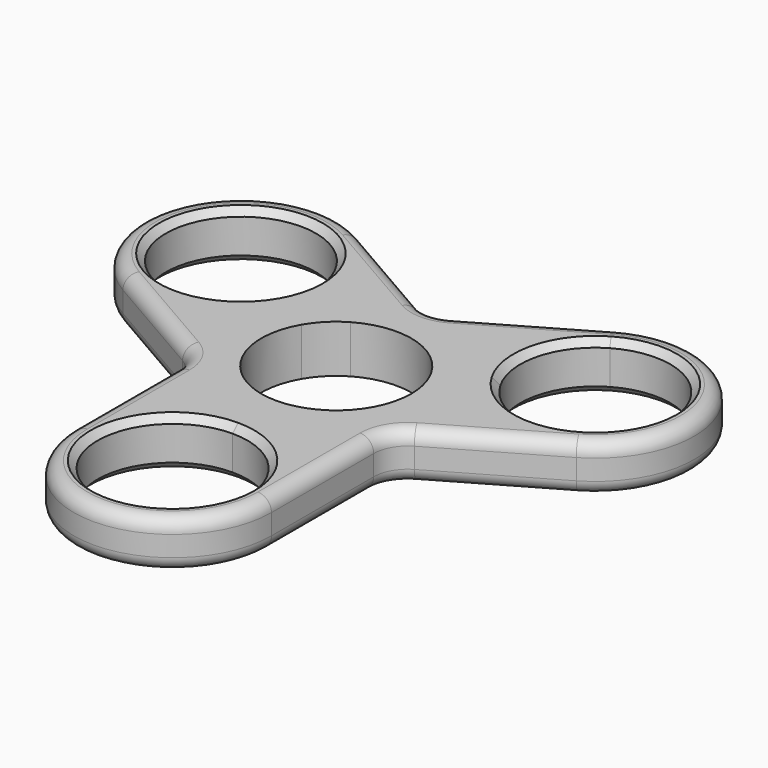
from build123d import *

# Parameters (mm, degrees)
F1_DEPTH    = 7
F3_DEPTH    = 7.001
F5_COUNT    = 3
F7_T1_DEPTH = 7
F8_R        = 2
F9_SIZE     = 1


# Not quite as in the source:
# - a fillet or chamfer that OpenCascade refuses, or shapes differently, is made with other operations: its cross-section is extruded or revolved along the edge and cut away or added
# - a feature names something its author has since deleted; it is built from what else it names


with BuildPart() as f1:
    # F0 (on Top) → F1 (new body)
    with BuildSketch(Plane.XY):
        with BuildLine():
            ThreePointArc((-14.5, 0), (0, -14.5), (14.5, 0))
            ThreePointArc((14.5, 0), (0, 14.5), (-14.5, 0))
        make_face()
        with BuildLine():
            Line((14.5, -30), (14.5, 0))
            ThreePointArc((14.5, 0), (0, -14.5), (-14.5, 0))
            Line((-14.5, 0), (-14.5, -30))
            ThreePointArc((-14.5, -30), (0, -15.5), (14.5, -30))
        make_face()
        with BuildLine():
            ThreePointArc((-14.5, -30), (0, -44.5), (14.5, -30))
            ThreePointArc((14.5, -30), (0, -15.5), (-14.5, -30))
        make_face()
    extrude(amount=F1_DEPTH)

    # F2 (on face) → F3 (cut, through all)
    with BuildSketch(Plane.XY.offset(7)):
        with BuildLine():
            ThreePointArc((0, -11), (7.7781745931, -7.7781745931), (11, 0))
            ThreePointArc((11, 0), (-7.7781745931, 7.7781745931), (0, -11))
        make_face()
        with BuildLine():
            ThreePointArc((11, -30), (7.7781745931, -22.2218254069), (0, -19))
            ThreePointArc((0, -19), (-7.7781745931, -37.7781745931), (11, -30))
        make_face()
    extrude(amount=-F3_DEPTH, mode=Mode.SUBTRACT)


with BuildPart() as f5_1:
    # F5: instance of F1
    add(f1.part.rotate(Axis((0, 0, 13.2415927947), (0, 0, 1)), 1 * 360 / F5_COUNT))


with BuildPart() as f5_2:
    # F5: instance of F1
    add(f1.part.rotate(Axis((0, 0, 13.2415927947), (0, 0, 1)), 2 * 360 / F5_COUNT))


with BuildPart() as f1_1:
    add(f1.part)

    # F6: union F5_2, F5_1
    add(f5_2.part)
    add(f5_1.part)

    # F7: fillet of radius 5 on 6 edges, made by hand

    # F7_s2 → F7_t1 (join)
    with BuildSketch(Plane.XY):
        with BuildLine():
            ThreePointArc((17, -6.9282032303), (15.1698729811, -8.7583302492), (14.5, -11.2583302492))
            Line((14.5, -11.2583302492), (14.5, -8.3715789032))
            Line((14.5, -8.3715789032), (17, -6.9282032303))
        make_face()
        with BuildLine():
            ThreePointArc((-2.5, 18.1865334795), (0, 17.5166604984), (2.5, 18.1865334795))
            Line((2.5, 18.1865334795), (0, 16.7431578065))
            Line((0, 16.7431578065), (-2.5, 18.1865334795))
        make_face()
        with BuildLine():
            ThreePointArc((-14.5, -11.2583302492), (-15.1698729811, -8.7583302492), (-17, -6.9282032303))
            Line((-17, -6.9282032303), (-14.5, -8.3715789032))
            Line((-14.5, -8.3715789032), (-14.5, -11.2583302492))
        make_face()
    extrude(amount=F7_T1_DEPTH)

    # F8
    f8_edges = [f1_1.edges().sort_by_distance(p)[0] for p in [
        (38.53813, 22.25, 7),
        (0, -44.5, 0),
        (-25.115381, -2.242786, 0),
        (-15.169873, -8.75833, 0),
        (-14.5, -20.629165, 0),
        (14.5, -20.629165, 0),
        (15.169873, -8.75833, 0),
        (25.115381, -2.242786, 0),
        (38.53813, 22.25, 0),
        (10.615381, 22.871951, 0),
        (0, 17.51666, 0),
        (-10.615381, 22.871951, 0),
        (-38.53813, 22.25, 0),
        (-25.115381, -2.242786, 7),
        (-14.5, -20.629165, 7),
        (0, -44.5, 7),
        (14.5, -20.629165, 7),
        (25.115381, -2.242786, 7),
        (10.615381, 22.871951, 7),
        (-10.615381, 22.871951, 7),
        (-38.53813, 22.25, 7),
        (-15.169873, -8.75833, 7),
        (15.169873, -8.75833, 7),
        (0, 17.51666, 7),
    ]]
    fillet(f8_edges, radius=F8_R)

    # F9
    f9_edges = [f1_1.edges().sort_by_distance(p)[0] for p in [
        (-35.507042, 20.5, 7),
        (0, -41, 7),
        (35.507042, 20.5, 7),
        (0, -41, 0),
        (35.507042, 20.5, 0),
        (-35.507042, 20.5, 0),
    ]]
    chamfer(f9_edges, length=F9_SIZE)


solid = f1_1.part
